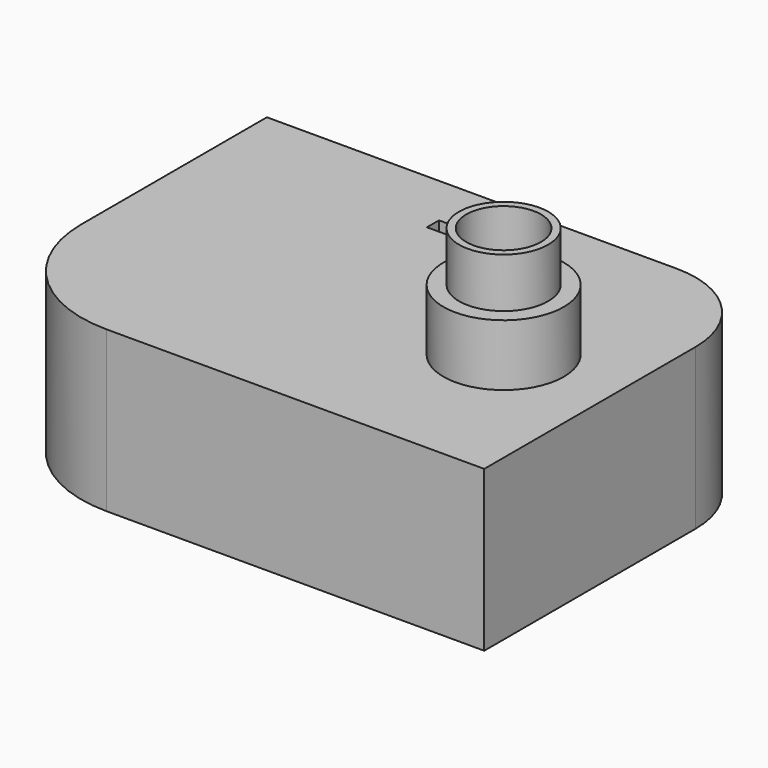
from build123d import *

# Parameters (mm, degrees)
F0_W      = 116.4761967957
F0_H      = 82.8055683523
F1_DEPTH  = 37
F2_R      = 13.9038489757
F3_DEPTH  = 14.2
F6_R      = 10.3135851835
F7_DEPTH  = 11.5
F8_R      = 8.6398790052
F9_DEPTH  = 33.5
F10_R     = 21.7279220614
F11_R     = 29.2119841047
F12_W     = 11.8597049732
F12_H     = 3.4746369347
F13_DEPTH = 25


# Not quite as in the source:
# - the program builds the solid bodies; features that only make, move or delete a surface that nothing else refers to are left out


with BuildPart() as f1:
    # F0 (on Top) → F1 (new body)
    with BuildSketch(Plane.XY):
        with Locations((0.5078110844, -10.3384470567)):
            Rectangle(F0_W, F0_H)
    extrude(amount=F1_DEPTH)

    # F2 (on face) → F3 (join)
    with BuildSketch(Plane.XY.offset(37)):
        with Locations((33.5578107329, -14.6564913073)):
            Circle(F2_R)
    extrude(amount=F3_DEPTH)

    # F6 (on face) → F7 (join)
    with BuildSketch(Plane.XY.offset(51.2)):
        with Locations((33.5578107329, -14.6564913073)):
            Circle(F6_R)
    extrude(amount=F7_DEPTH)

    # F8 (on face) → F9 (cut)
    with BuildSketch(Plane.XY.offset(62.7)):
        with Locations((33.5578107329, -14.6564913073)):
            Circle(F8_R)
    extrude(amount=-F9_DEPTH, mode=Mode.SUBTRACT)

    # F10
    f10_edges = [f1.edges().sort_by_distance(p)[0] for p in [
        (58.745909, 31.064337, 18.5),
    ]]
    fillet(f10_edges, radius=F10_R)

    # F11
    f11_edges = [f1.edges().sort_by_distance(p)[0] for p in [
        (-57.730287, -51.741231, 18.5),
    ]]
    fillet(f11_edges, radius=F11_R)

    # F12 (on face) → F13 (cut)
    with BuildSketch(Plane.XY.offset(37)):
        with Locations((-2.380865044, 17.2674548812)):
            Rectangle(F12_W, F12_H)
    extrude(amount=-F13_DEPTH, mode=Mode.SUBTRACT)


solid = f1.part
